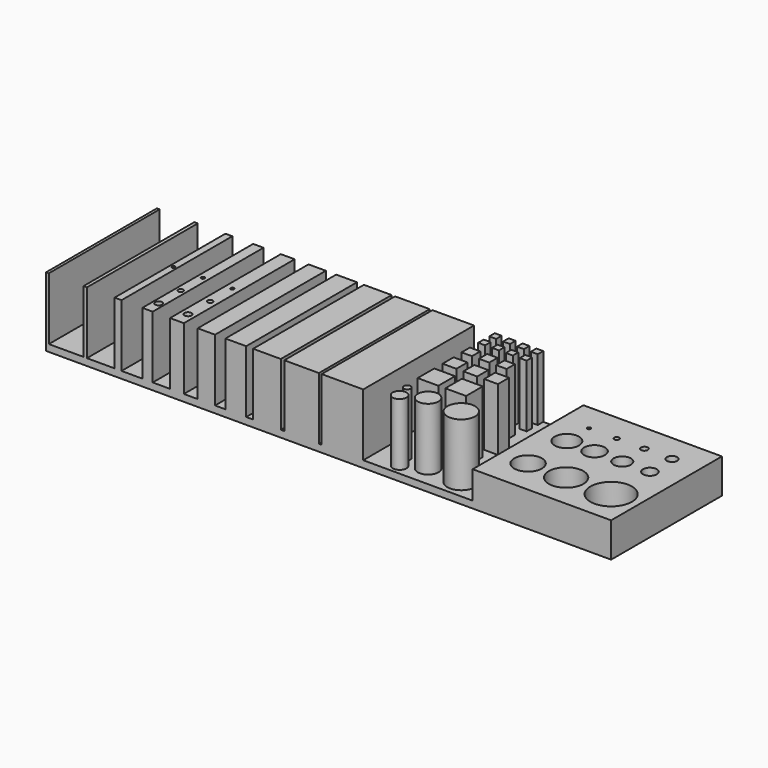
from build123d import *

# Parameters (mm, degrees)
F0_W          = 81.6
F0_H          = 20
F1_DEPTH      = 1
F2_W          = 0.4
F2_H          = 20
F2_W_2        = 0.5
F2_W_3        = 1
F2_W_4        = 1.5
F2_W_5        = 2
F2_W_6        = 2.5
F2_W_7        = 3
F2_W_8        = 4
F2_W_9        = 5
F2_W_10       = 6
F2_H_2        = 1
F2_H_3        = 1.5
F2_H_4        = 2
F2_H_5        = 3
F2_R          = 0.5
F2_R_2        = 1
F2_R_3        = 1.5
F2_R_4        = 2
F3_DEPTH      = 9
F4_W          = 19.9949190378
F4_H          = 20
F5_DEPTH      = 4
F6_R          = 0.25
F7_DEPTH      = 10.001
F8_R          = 0.25
F8_R_2        = 0.375
F8_R_3        = 0.5
F9_DEPTH      = 10.001
F10_R         = 0.25
F10_R_2       = 0.375
F10_R_3       = 0.5
F11_DEPTH     = 10.001
F12_R         = 3
F12_R_2       = 0.5
F12_R_3       = 2
F12_R_4       = 1
F12_R_5       = 1.75
F12_R_6       = 0.25
F12_R_7       = 0.375
F12_R_8       = 1.5
F12_R_9       = 0.75
F12_R_10      = 1.25
F12_R_11      = 2.5
F13_DEPTH     = 5.001
F14_TEXT_SIZE = 3.4722222222
F15_DEPTH     = 1


# Not quite as in the source:
# - Text() gives the source's letters only with a copy of the font that has no kerning and outlines rounded to 1/6400 em; it was checked with that copy


with BuildPart() as f1:
    # F0 (on Top) → F1 (new body)
    with BuildSketch(Plane.XY):
        with Locations((40.8, 10)):
            Rectangle(F0_W, F0_H)
    extrude(amount=F1_DEPTH)

    # F2 (on face) → F3 (join)
    with BuildSketch(Plane.XY.offset(1)):
        with Locations((0.2, 10)):
            Rectangle(F2_W, F2_H)
        with Locations((5.65, 10)):
            Rectangle(F2_W_2, F2_H)
        with Locations((10.4, 10)):
            Rectangle(F2_W_3, F2_H)
        with Locations((14.65, 10)):
            Rectangle(F2_W_4, F2_H)
        with Locations((18.9, 10)):
            Rectangle(F2_W_5, F2_H)
        with Locations((23.15, 10)):
            Rectangle(F2_W_6, F2_H)
        with Locations((27.4, 10)):
            Rectangle(F2_W_7, F2_H)
        with Locations((31.9, 10)):
            Rectangle(F2_W_8, F2_H)
        with Locations((36.9, 10)):
            Rectangle(F2_W_9, F2_H)
        with Locations((42.8, 10)):
            Rectangle(F2_W_10, F2_H)
        with Locations((49.3, 17.5)):
            Rectangle(F2_W_3, F2_H_2)
        with Locations((49.3, 19.5)):
            Rectangle(F2_W_3, F2_H_2)
        with Locations((51.3, 19.5)):
            Rectangle(F2_W_3, F2_H_2)
        with Locations((53.3, 19.5)):
            Rectangle(F2_W_3, F2_H_2)
        with Locations((55.3, 19.5)):
            Rectangle(F2_W_3, F2_H_2)
        with Locations((55.3, 17.5)):
            Rectangle(F2_W_3, F2_H_2)
        with Locations((53.3, 17.5)):
            Rectangle(F2_W_3, F2_H_2)
        with Locations((51.3, 17.5)):
            Rectangle(F2_W_3, F2_H_2)
        with Locations((49.55, 14.75)):
            Rectangle(F2_W_4, F2_H_3)
        with Locations((52.05, 14.75)):
            Rectangle(F2_W_4, F2_H_3)
        with Locations((54.55, 14.75)):
            Rectangle(F2_W_4, F2_H_3)
        with Locations((49.8560581097, 11.5)):
            Rectangle(F2_W_5, F2_H_4)
        with Locations((52.8560581097, 11.5)):
            Rectangle(F2_W_5, F2_H_4)
        with Locations((55.8560581097, 11.5)):
            Rectangle(F2_W_5, F2_H_4)
        with Locations((50.3560581097, 7.5)):
            Rectangle(F2_W_7, F2_H_5)
        with Locations((54.3560581097, 7.5)):
            Rectangle(F2_W_7, F2_H_5)
        with Locations((49.3560581097, 3.5)):
            Circle(F2_R)
        with Locations((49.8560581097, 1.5)):
            Circle(F2_R_2)
        with Locations((52.7678541839, 3)):
            Circle(F2_R_3)
        with Locations((57.7678541839, 2.738554962)):
            Circle(F2_R_4)
    extrude(amount=F3_DEPTH)

    # F4 (on face) → F5 (join)
    with BuildSketch(Plane.XY.offset(1)):
        with Locations((71.6025404811, 10)):
            Rectangle(F4_W, F4_H)
    extrude(amount=F5_DEPTH)

    # F6 (on face) → F7 (cut, through all)
    with BuildSketch(Plane.XY.offset(10)):
        with Locations((10.4, 10)):
            Circle(F6_R)
    extrude(amount=-F7_DEPTH, mode=Mode.SUBTRACT)

    # F8 (on face) → F9 (cut, through all)
    with BuildSketch(Plane.XY.offset(10)):
        with Locations((14.65, 10)):
            Circle(F8_R)
        with Locations((14.65, 6)):
            Circle(F8_R_2)
        with Locations((14.65, 2)):
            Circle(F8_R_3)
    extrude(amount=-F9_DEPTH, mode=Mode.SUBTRACT)

    # F10 (on face) → F11 (cut, through all)
    with BuildSketch(Plane.XY.offset(10)):
        with Locations((18.9, 10)):
            Circle(F10_R)
        with Locations((18.9, 6)):
            Circle(F10_R_2)
        with Locations((18.9, 2)):
            Circle(F10_R_3)
    extrude(amount=-F11_DEPTH, mode=Mode.SUBTRACT)

    # F12 (on face) → F13 (cut, through all)
    with BuildSketch(Plane.XY.offset(5)):
        with Locations((77.6050809622, 5)):
            Circle(F12_R)
        with Locations((73.6050809622, 16)):
            Circle(F12_R_2)
        with Locations((65.6050809622, 5)):
            Circle(F12_R_3)
        with Locations((77.6050809622, 12)):
            Circle(F12_R_4)
        with Locations((65.6050809622, 12)):
            Circle(F12_R_5)
        with Locations((65.6050809622, 16)):
            Circle(F12_R_6)
        with Locations((69.6050809622, 16)):
            Circle(F12_R_7)
        with Locations((69.6050809622, 12)):
            Circle(F12_R_8)
        with Locations((77.6050809622, 16)):
            Circle(F12_R_9)
        with Locations((73.6050809622, 12)):
            Circle(F12_R_10)
        with Locations((71.1050809622, 5)):
            Circle(F12_R_11)
    extrude(amount=-F13_DEPTH, mode=Mode.SUBTRACT)

    # F14 (on face) → F15 (join)
    with BuildSketch(Plane.XY.offset(1)):
        with Locations((58.3279110235, 6.5)):
            Text('4', F14_TEXT_SIZE, font='Open Sans', text_align=(TextAlign.LEFT, TextAlign.BOTTOM))
        with Locations((58.3279110235, 10)):
            Text('3', F14_TEXT_SIZE, font='Open Sans', text_align=(TextAlign.LEFT, TextAlign.BOTTOM))
        with Locations((58.1214223082, 17)):
            Text('1', F14_TEXT_SIZE, font='Open Sans', text_align=(TextAlign.LEFT, TextAlign.BOTTOM))
        with Locations((58.3279110235, 13.5)):
            Text('2', F14_TEXT_SIZE, font='Open Sans', text_align=(TextAlign.LEFT, TextAlign.BOTTOM))
    extrude(amount=F15_DEPTH)


solid = f1.part
